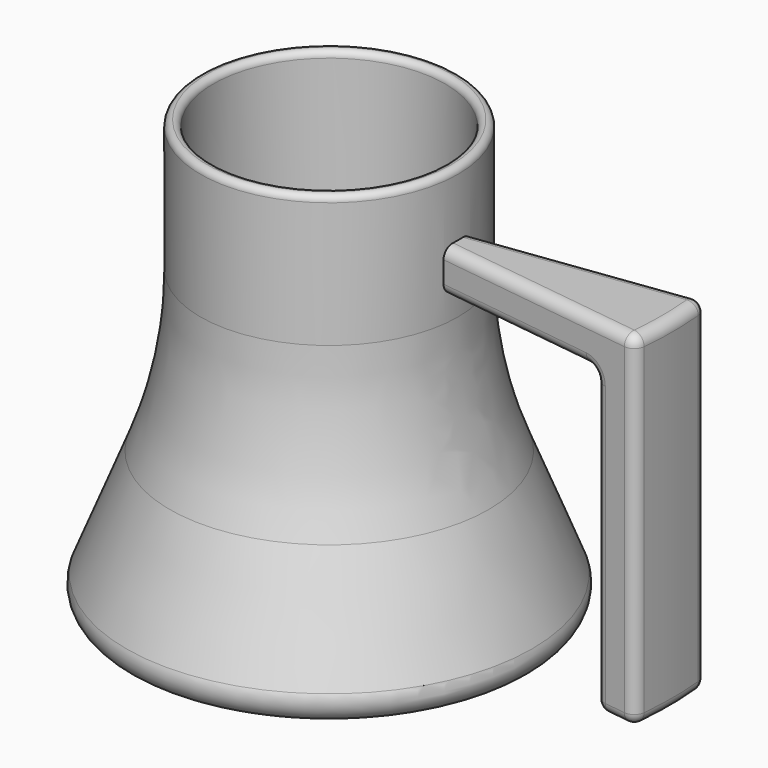
from build123d import *

# Parameters (mm, degrees)
F0_R          = 50
F2_R          = 30
F4_DEPTH      = 50
F5_T          = -3
F6_R          = 1.49999
F7_R          = 5
F9_ANGLE_BACK = 7.5
F9_ANGLE      = 15
F10_R         = 2.5
F11_R         = 100


# Not quite as in the source:
# - a fillet or chamfer is up to 0.001 mm smaller than in the source, because OpenCascade refuses the exact size


with BuildPart() as f3:
    # F0 (on Top) → F3 section 0
    with BuildSketch(Plane.XY):
        Circle(F0_R)
    # F2 (on offset) → F3 section 1
    with BuildSketch(Plane.XY.offset(50)):
        Circle(F2_R)
    loft()

    # F4 (add): a face of the model
    f4_faces = [f3.faces().sort_by_distance(p)[0] for p in [
        (0, 0, 50),
    ]]
    extrude(f4_faces, amount=F4_DEPTH)

    # F5
    f5_openings = [f3.faces().sort_by_distance(p)[0] for p in [
        (0, 0, 100),
    ]]
    offset(amount=F5_T, openings=f5_openings, kind=Kind.INTERSECTION)

    # F6 (radius 1.5 in the source; OpenCascade refuses exactly that, so slightly less here)
    f6_edges = [f3.edges().sort_by_distance(p)[0] for p in [
        (-30, 0, 100),
        (-27, 0, 100),
    ]]
    fillet(f6_edges, radius=F6_R)

    # F7
    f7_edges = [f3.edges().sort_by_distance(p)[0] for p in [
        (-50, 0, 0),
        (-45.568901, 0, 3),
    ]]
    fillet(f7_edges, radius=F7_R)

    # F8 (on Front) → F9 (revolve)
    with BuildSketch(Plane.XZ, mode=Mode.PRIVATE) as f9_sk:
        Polygon((30, 85), (30, 80), (30, 75), (70, 75), (70, 5), (80, 5), (80, 85), align=None)
    revolve(f9_sk.sketch.rotate(Axis((0, 0, 40), (0, 0, -1)), -F9_ANGLE_BACK), axis=Axis((0, 0, 40), (0, 0, -1)), revolution_arc=F9_ANGLE)

    # F10
    f10_edges = [f3.edges().sort_by_distance(p)[0] for p in [
        (54.529467, -7.178941, 85),
        (54.529467, 7.178941, 85),
        (79.315589, 10.442095, 45),
        (79.315589, -10.442095, 45),
        (80, 0, 85),
        (80, 0, 5),
        (74.358365, 9.789464, 5),
        (74.358365, -9.789464, 5),
        (69.40114, 9.136833, 40),
        (69.40114, -9.136833, 40),
        (49.572243, 6.52631, 75),
        (49.572243, -6.52631, 75),
        (70, 0, 5),
        (70, 0, 75),
    ]]
    fillet(f10_edges, radius=F10_R)

    # F11
    f11_edges = [f3.edges().sort_by_distance(p)[0] for p in [
        (-30, 0, 50),
        (-27, 0, 49.422253),
    ]]
    fillet(f11_edges, radius=F11_R)


solid = f3.part
